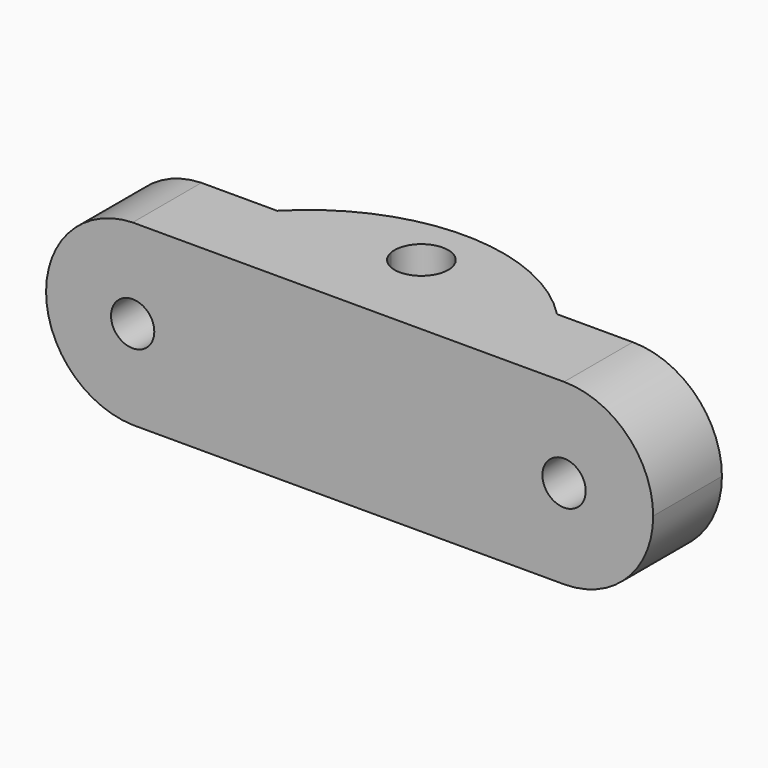
from build123d import *
from build123d import SkipClean  # not in build123d's __all__

# Parameters (mm, degrees)
F1_DEPTH      = 8
F3_DEPTH      = 8.2965155193
F3_DEPTH_BACK = 8.2965155193
F4_R          = 2.5
F5_DEPTH      = 12.5


with BuildPart() as f1:
    # F0 (on Front) → F1 (new body)
    with BuildSketch(Plane.XZ):
        with BuildLine():
            Line((20.0802286013, 8.2965155193), (-20.0802286013, 8.2965155193))
            ThreePointArc((-20.0802286013, 8.2965155193), (-25.7931508501, 5.7833391211), (-28.1397494181, 0))
            Line((-28.1397494181, 0), (-22.0952286013, 0))
            ThreePointArc((-22.0952286013, 0), (-20.0802286013, 2.015), (-18.0652286013, 0))
            Line((-18.0652286013, 0), (18.0652286013, 0))
            ThreePointArc((18.0652286013, 0), (20.0802286013, 2.015), (22.0952286013, 0))
            Line((22.0952286013, 0), (28.3767441206, 0))
            ThreePointArc((28.3767441206, 0), (25.9467509852, 5.8665223839), (20.0802286013, 8.2965155193))
        make_face()
        with BuildLine():
            Line((-22.0952286013, 0), (-28.1397494181, 0))
            ThreePointArc((-28.1397494181, 0), (-25.7931508501, -5.7833391211), (-20.0802286013, -8.2965155193))
            Line((-20.0802286013, -8.2965155193), (20.0802286013, -8.2965155193))
            ThreePointArc((20.0802286013, -8.2965155193), (25.9467509852, -5.8665223839), (28.3767441206, 0))
            Line((28.3767441206, 0), (22.0952286013, 0))
            ThreePointArc((22.0952286013, 0), (20.0802286013, -2.015), (18.0652286013, 0))
            Line((18.0652286013, 0), (-18.0652286013, 0))
            ThreePointArc((-18.0652286013, 0), (-20.0802286013, -2.015), (-22.0952286013, 0))
        make_face()
    extrude(amount=F1_DEPTH)

    # F2 (on Top) → F3 (join, two sides)
    with BuildSketch(Plane.XY) as f3_sk:
        with BuildLine():
            Line((2.4494897428, 0), (13.0258305651, 0))
            ThreePointArc((13.0258305651, 0), (0, 5.5), (-13.0258305651, 0))
            Line((-13.0258305651, 0), (-2.4494897428, 0))
            ThreePointArc((-2.4494897428, 0), (-0.251272405, 2.9873403825), (2.5, 0.5))
            ThreePointArc((2.5, 0.5), (2.4873403825, 0.248727595), (2.4494897428, 0))
        make_face()
    extrude(amount=F3_DEPTH)
    extrude(f3_sk.sketch, amount=-F3_DEPTH_BACK)

    # F4 (on Top) → F5 (cut, symmetric)
    with BuildSketch(Plane.XY):
        with Locations((0, 0.5)):
            Circle(F4_R)
    with SkipClean():  # cleaning this boolean's faces spoils the solid; the shape is the same uncleaned
        extrude(amount=F5_DEPTH, both=True, mode=Mode.SUBTRACT)


solid = f1.part
